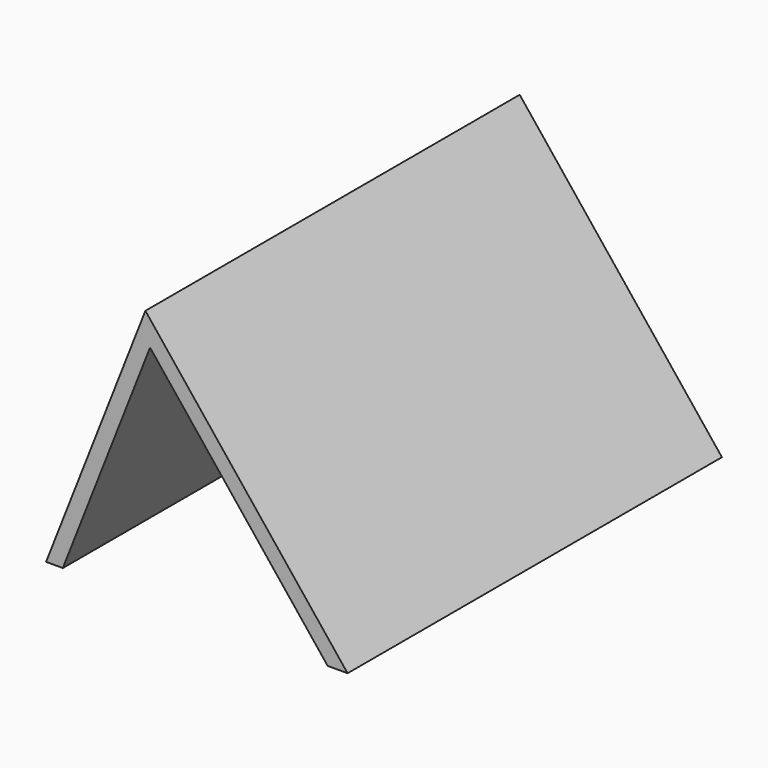
from build123d import *

# Parameters (mm, degrees)
F1_DEPTH = 22.5


# Not quite as in the source:
# - a feature of the source that left no trace in its solid (it failed there, or was rolled back) is left out


with BuildPart() as f1:
    # F0 (on Front) → F1 (new body, symmetric)
    with BuildSketch(Plane.XZ):
        Polygon((-0.4483525125, 24.3668013383), (-10, 0), (-8.3888718351, 0), (0, 21.4004938652), (17.0807954173, 0), (19, 0), align=None)
    extrude(amount=F1_DEPTH, both=True)


solid = f1.part
